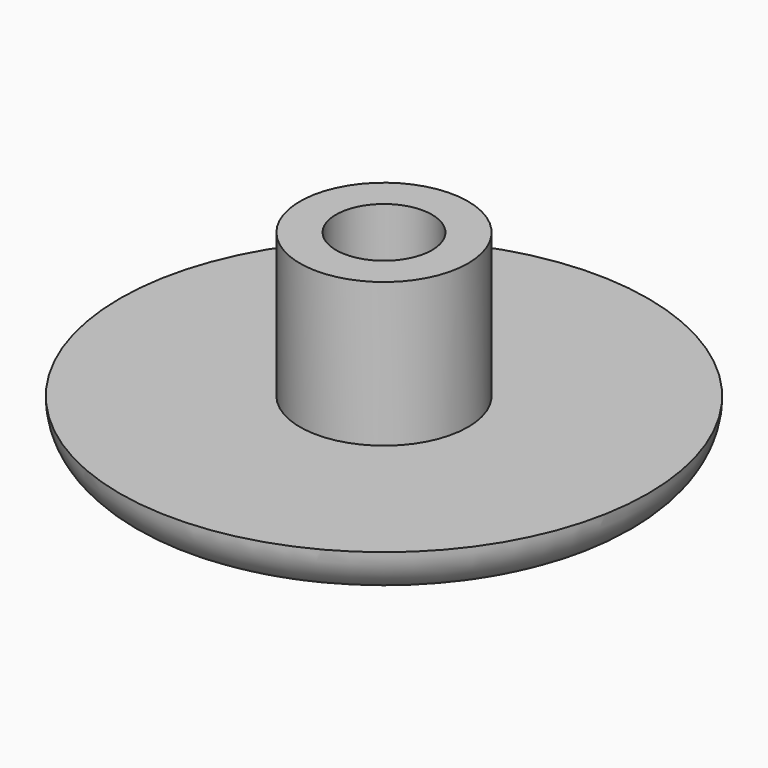
from build123d import *

# Parameters (mm, degrees)
F0_R     = 11
F1_DEPTH = 2
F2_R     = 3.5
F3_DEPTH = 6
F4_R     = 2
F5_DEPTH = 6
F6_R     = 1.99999


# Not quite as in the source:
# - a fillet or chamfer is up to 0.001 mm smaller than in the source, because OpenCascade refuses the exact size


with BuildPart() as f1:
    # F0 (on Top) → F1 (new body)
    with BuildSketch(Plane.XY):
        Circle(F0_R)
    extrude(amount=F1_DEPTH)

    # F2 (on face) → F3 (join)
    with BuildSketch(Plane.XY.offset(2)):
        Circle(F2_R)
    extrude(amount=F3_DEPTH)

    # F4 (on face) → F5 (cut)
    with BuildSketch(Plane.XY.offset(8)):
        Circle(F4_R)
    extrude(amount=-F5_DEPTH, mode=Mode.SUBTRACT)

    # F6 (radius 2 in the source; OpenCascade refuses exactly that, so slightly less here)
    f6_edges = [f1.edges().sort_by_distance(p)[0] for p in [
        (-11, 0, 0),
    ]]
    fillet(f6_edges, radius=F6_R)


solid = f1.part
